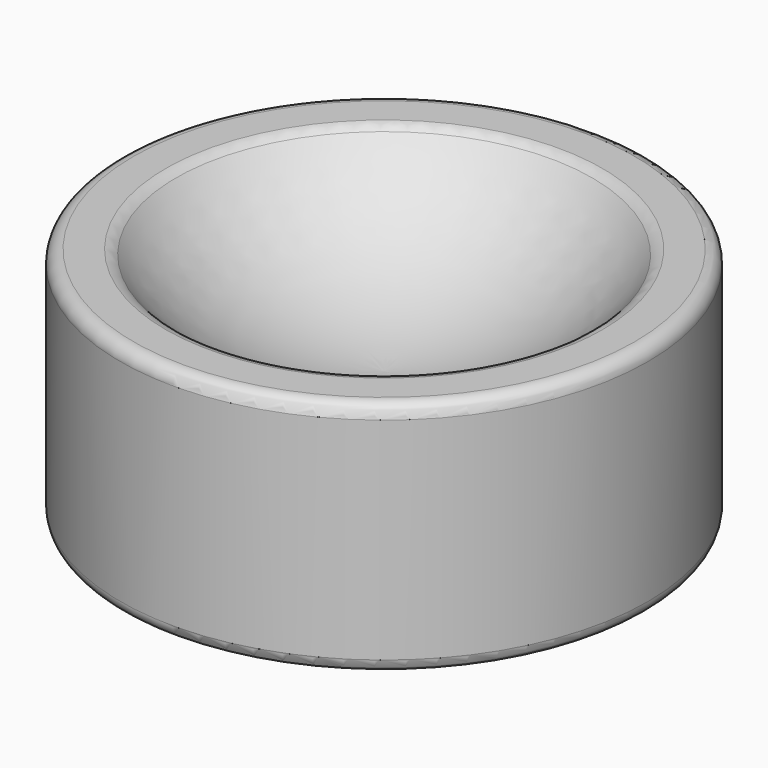
from build123d import *

# Parameters (mm, degrees)
F2_R     = 2.5
F3_DEPTH = 1
F4_R     = 2.5
F5_DEPTH = 4
F6_R     = 0.49999
F7_R     = 0.5


# Not quite as in the source:
# - a fillet or chamfer is up to 0.001 mm smaller than in the source, because OpenCascade refuses the exact size


with BuildPart() as f1:
    # F0 (on Front) → F1 (revolve)
    with BuildSketch(Plane.XZ):
        with BuildLine():
            Line((10, -6), (8.0299019418, -6))
            ThreePointArc((8.0299019418, -6), (4.4755477951, -8.9483166731), (0, -10.0865067004))
            Line((0, -10.0865067004), (0, -15))
            Line((0, -15), (10, -15))
            Line((10, -15), (10, -6))
        make_face()
    revolve(axis=Axis((0, 0, -12.5432533502), (0, 0, 1)))

    # F2 (on face) → F3 (cut)
    with BuildSketch(Plane(origin=(0, 0, -15), x_dir=(1, 0, 0), z_dir=(0, 0, -1))):
        Circle(F2_R)
    extrude(amount=-F3_DEPTH, mode=Mode.SUBTRACT)

    # F4 (on face) → F5 (cut)
    with BuildSketch(Plane(origin=(0, 0, -15), x_dir=(1, 0, 0), z_dir=(0, 0, -1))):
        with Locations((-5.1961524227, 3)):
            Circle(F4_R)
        with Locations((0, 6)):
            Circle(F4_R)
        with Locations((5.1961524227, 3)):
            Circle(F4_R)
        with Locations((5.1961524227, -3)):
            Circle(F4_R)
        with Locations((0, -6)):
            Circle(F4_R)
        with Locations((-5.1961524227, -3)):
            Circle(F4_R)
    extrude(amount=-F5_DEPTH, mode=Mode.SUBTRACT)

    # F6 (radius 0.5 in the source; OpenCascade refuses exactly that, so slightly less here)
    f6_edges = [f1.edges().sort_by_distance(p)[0] for p in [
        (2.696152, 3, -15),
        (-2.5, 6, -15),
        (-7.696152, 3, -15),
        (-7.696152, -3, -15),
        (-2.5, -6, -15),
        (2.696152, -3, -15),
        (2.696152, 3, -11),
        (-2.5, 6, -11),
        (-7.696152, 3, -11),
        (-7.696152, -3, -11),
        (-2.5, -6, -11),
        (2.696152, -3, -11),
    ]]
    fillet(f6_edges, radius=F6_R)

    # F7
    f7_edges = [f1.edges().sort_by_distance(p)[0] for p in [
        (-10, 0, -15),
        (-10, 0, -6),
        (-8.029902, 0, -6),
    ]]
    fillet(f7_edges, radius=F7_R)


solid = f1.part
